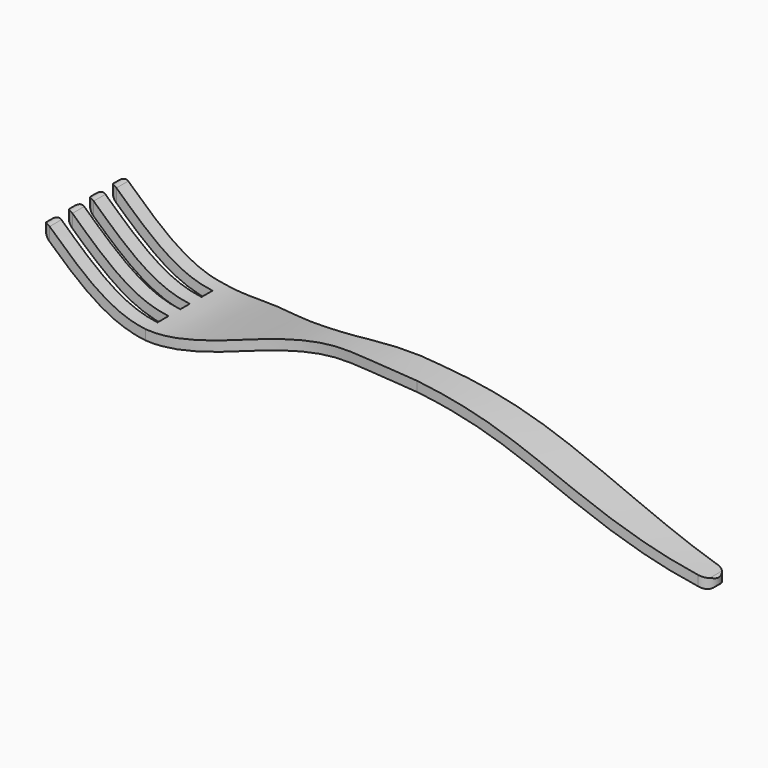
from build123d import *

# Parameters (mm, degrees)
F1_DEPTH      = 25.4
F2_W          = 179.1693205014
F2_H          = 43.9865416847
F3_DEPTH      = 100.584
F3_DEPTH_BACK = 27.432


# Not quite as in the source:
# - the dataset's text gives a spline's control points without its knots; the knots are read off the source's solid


with BuildPart() as f1:
    # F0 (on Front) → F1 (new body)
    with BuildSketch(Plane.XZ):
        with BuildLine():
            add(Edge.make_bspline(
                [(0, 0), (4.3641683055, -4.0051600351), (13.1746485591, -12.1785269438), (29.2498095353, -17.9432029217), (60.9537254972, -7.8903386303), (98.3671771263, -9.9596926847), (122.8718833311, -17.9427951784), (147.1825008774, -28.7291969767), (162.035150421, -31.6641757833)],
                knots=[0, 0, 0, 0, 0.1333019949, 0.258773735, 0.4401505179, 0.633884626, 0.7949050626, 1, 1, 1, 1], degree=3))
            ThreePointArc((0, 0), (-1.7944010964, -0.0769721067), (-1.7174289897, -1.8713732031))
            add(Edge.make_bspline(
                [(-1.7174289897, -1.8713732031), (0.3254704589, -3.7462182262), (4.535458283, -7.6309070127), (11.2480115862, -12.9533694797), (17.2738853397, -16.1840756852), (22.7362354977, -17.6662598971), (26.4572800642, -18.0684830642), (29.6577070125, -18.0488658662), (32.1397483087, -17.8740243865), (34.7021089418, -17.5705107004), (38.2218305862, -17.0260081066), (42.8052188526, -16.1426166242), (48.5524018525, -14.935604403), (53.4968100578, -13.9504578037), (57.5115334385, -13.2592868054), (60.5413955786, -12.8098827746), (63.5870850754, -12.4510490837), (67.6803417482, -12.0895437553), (72.81856179, -11.8472534431), (78.9330801778, -11.8616784998), (84.9060461356, -12.149886523), (89.6914786304, -12.591508326), (93.359411922, -13.0491806905), (96.0195275612, -13.440550157), (98.5746135007, -13.8752285116), (101.8428850677, -14.5099951096), (105.7274834353, -15.4129636803), (110.2312106044, -16.6881126685), (114.7425216387, -18.1739630326), (118.6417643625, -19.6034632062), (121.9216921708, -20.8701211638), (125.3359263851, -22.2213984095), (129.8436621661, -24.0356189643), (135.6012085624, -26.3075074614), (141.6753631862, -28.5686907701), (150.1569808546, -31.4284179292), (156.9066682104, -33.2398712545), (161.5427517348, -34.1559910923)],
                knots=[0, 0, 0, 0, 0.0625, 0.125, 0.1875, 0.21875, 0.25, 0.265625, 0.28125, 0.296875, 0.3125, 0.34375, 0.375, 0.40625, 0.421875, 0.4375, 0.453125, 0.46875, 0.5, 0.53125, 0.5625, 0.59375, 0.609375, 0.625, 0.640625, 0.65625, 0.6875, 0.71875, 0.75, 0.78125, 0.796875, 0.8125, 0.84375, 0.875, 0.90625, 0.9375, 1, 1, 1, 1], degree=3))
            ThreePointArc((161.5427517348, -34.1559910923), (163.0348587324, -33.1562827809), (162.035150421, -31.6641757833))
        make_face()
    extrude(amount=F1_DEPTH)

    # F2 (on Top) → F3 (cut, two sides)
    with BuildSketch(Plane.XY) as f3_sk:
        with Locations((83.3395454101, -12.7)):
            Rectangle(F2_W, F2_H)
        with BuildLine():
            ThreePointArc((0, -3.81), (-1.905, -1.905), (0, 0))
            add(Edge.make_bspline(
                [(0, 0), (5.938945419, 0.1487556476), (16.5227470311, 0.6150495786), (24.8320070622, 0)],
                knots=[0, 0, 0, 0, 0.2380062526, 0.2380062526, 0.2380062526, 0.2380062526], degree=3))
            add(Edge.make_bspline(
                [(24.8320070622, 0), (31.7539464423, -0.5123604127), (41.5119426085, -2.8183422934), (52.413871511, -8.0831416139), (67.517929997, -10.7861502317), (76.6360313396, -8.119793766), (88.1742686033, -8.5318738128)],
                knots=[0.2380062526, 0.2380062526, 0.2380062526, 0.2380062526, 0.4362747923, 0.6000722231, 0.7740495288, 1, 1, 1, 1], degree=3))
            add(Edge.make_bspline(
                [(88.1742686033, -8.5318738128), (122.1121549606, -7.7734852675), (133.3644173663, -7.1712665693), (159.8452329636, -9.6694547683)],
                knots=[0, 0, 0, 0, 71.6799917882, 71.6799917882, 71.6799917882, 71.6799917882], degree=3))
            ThreePointArc((159.8452329636, -9.6694547683), (162.7722692296, -12.7), (159.8452329636, -15.7305452317))
            add(Edge.make_bspline(
                [(88.1742686033, -16.8681261872), (122.1121549606, -17.6265147325), (133.3644173663, -18.2287334307), (159.8452329636, -15.7305452317)],
                knots=[0, 0, 0, 0, 71.6799917882, 71.6799917882, 71.6799917882, 71.6799917882], degree=3))
            add(Edge.make_bspline(
                [(24.8320070622, -25.4), (31.7539464423, -24.8876395873), (41.5119426085, -22.5816577066), (52.413871511, -17.3168583861), (67.517929997, -14.6138497683), (76.6360313396, -17.280206234), (88.1742686033, -16.8681261872)],
                knots=[0.2380062526, 0.2380062526, 0.2380062526, 0.2380062526, 0.4362747923, 0.6000722231, 0.7740495288, 1, 1, 1, 1], degree=3))
            add(Edge.make_bspline(
                [(0, -25.4), (5.938945419, -25.5487556476), (16.5227470311, -26.0150495786), (24.8320070622, -25.4)],
                knots=[0, 0, 0, 0, 0.2380062526, 0.2380062526, 0.2380062526, 0.2380062526], degree=3))
            ThreePointArc((0, -25.4), (-1.905, -23.495), (0, -21.59))
            Line((0, -21.59), (24.8320070622, -21.59))
            Line((24.8320070622, -21.59), (24.8320070622, -18.034))
            Line((24.8320070622, -18.034), (0, -18.034))
            ThreePointArc((0, -18.034), (-1.905, -16.129), (0, -14.224))
            Line((0, -14.224), (24.8320070622, -14.224))
            Line((24.8320070622, -14.224), (24.8320070622, -12.7))
            Line((24.8320070622, -12.7), (24.8320070622, -11.176))
            Line((24.8320070622, -11.176), (0, -11.176))
            ThreePointArc((0, -11.176), (-1.905, -9.271), (0, -7.366))
            Line((0, -7.366), (24.8320070622, -7.366))
            Line((24.8320070622, -7.366), (24.8320070622, -3.81))
            Line((24.8320070622, -3.81), (0, -3.81))
        make_face(mode=Mode.SUBTRACT)
    extrude(amount=-F3_DEPTH, mode=Mode.SUBTRACT)
    extrude(f3_sk.sketch, amount=F3_DEPTH_BACK, mode=Mode.SUBTRACT)


solid = f1.part
